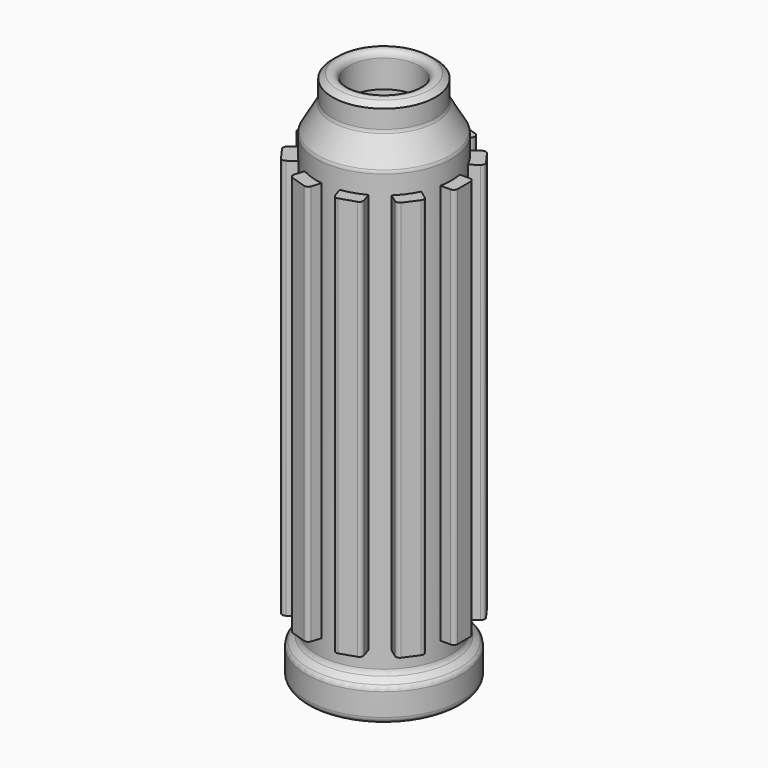
from build123d import *

# Parameters (mm, degrees)
F2_R            = 1.6
F4_W            = 6
F4_H            = 100
F5_COPIES_COUNT = 10
F6_R            = 1
F6_2_R          = 1
F6_3_R          = 1
F6_4_R          = 1
F6_5_R          = 1
F6_6_R          = 1
F6_7_R          = 1
F6_8_R          = 1
F6_9_R          = 1
F6_10_R         = 1


# Not quite as in the source:
# - a feature of the source that left no trace in its solid (it failed there, or was rolled back) is left out
# - a pattern or mirror of a feature is missing from the dataset's text; its kind, count and spacing are read off the source's solid


with BuildPart() as f1:
    # F0 (on Front) → F1 (revolve)
    with BuildSketch(Plane.XZ):
        with BuildLine():
            Line((10.75, 125), (10.75, 0))
            Line((10.75, 0), (19.325, 0))
            Line((19.325, 0), (19.325, 8))
            Line((19.325, 8), (16.7893237613, 10.1276849967))
            Line((16.7893237613, 10.1276849967), (16.7893237613, 120.1276849967))
            Line((16.7893237613, 120.1276849967), (12.8215908442, 127))
            Line((12.8215908442, 127), (12.8215908442, 132))
            ThreePointArc((12.8215908442, 132), (10.860884629, 133.5551954835), (8.8174703872, 135))
            Line((8.8174703872, 135), (8.8174703872, 125))
            Line((8.8174703872, 125), (10.75, 125))
        make_face()
    revolve(axis=Axis((0, 0, 18.1783709021), (0, 0, 1)))

    # F2
    f2_edges = [f1.edges().sort_by_distance(p)[0] for p in [
        (-8.81747, 0, 135),
        (-12.821591, 0, 127),
        (-16.789324, 0, 120.127685),
        (-16.789324, 0, 10.127685),
        (-19.325, 0, 8),
        (-19.325, 0, 0),
    ]]
    fillet(f2_edges, radius=F2_R)


with BuildPart() as f5:
    # F4 (on offset) → F5 (new body, up to the next surface of F1)
    with BuildSketch(Plane.YZ.offset(20)):
        with Locations((0, 65)):
            Rectangle(F4_W, F4_H)
    extrude(until=Until.NEXT, target=f1.part, dir=(-1, 0, 0))


with BuildPart() as f5_copies_1:
    # F5_copies: instance of F5
    add(f5.part.rotate(Axis((0, 0, 0), (0, 0, 1)), 1 * 360 / F5_COPIES_COUNT))

    # F6#2
    f6_2_edges = [f5_copies_1.edges().sort_by_distance(p)[0] for p in [
        (17.943696, 9.328654, 65),
        (14.416984, 14.182756, 65),
    ]]
    fillet(f6_2_edges, radius=F6_2_R)


with BuildPart() as f5_copies_2:
    # F5_copies: instance of F5
    add(f5.part.rotate(Axis((0, 0, 0), (0, 0, 1)), 2 * 360 / F5_COPIES_COUNT))

    # F6#3
    f6_3_edges = [f5_copies_2.edges().sort_by_distance(p)[0] for p in [
        (9.033509, 18.094079, 65),
        (3.32717, 19.948181, 65),
    ]]
    fillet(f6_3_edges, radius=F6_3_R)


with BuildPart() as f5_copies_3:
    # F5_copies: instance of F5
    add(f5.part.rotate(Axis((0, 0, 0), (0, 0, 1)), 3 * 360 / F5_COPIES_COUNT))

    # F6#4
    f6_4_edges = [f5_copies_3.edges().sort_by_distance(p)[0] for p in [
        (-3.32717, 19.948181, 65),
        (-9.033509, 18.094079, 65),
    ]]
    fillet(f6_4_edges, radius=F6_4_R)


with BuildPart() as f5_copies_4:
    # F5_copies: instance of F5
    add(f5.part.rotate(Axis((0, 0, 0), (0, 0, 1)), 4 * 360 / F5_COPIES_COUNT))

    # F6#5
    f6_5_edges = [f5_copies_4.edges().sort_by_distance(p)[0] for p in [
        (-14.416984, 14.182756, 65),
        (-17.943696, 9.328654, 65),
    ]]
    fillet(f6_5_edges, radius=F6_5_R)


with BuildPart() as f5_copies_5:
    # F5_copies: instance of F5
    add(f5.part.rotate(Axis((0, 0, 0), (0, 0, 1)), 5 * 360 / F5_COPIES_COUNT))

    # F6#6
    f6_6_edges = [f5_copies_5.edges().sort_by_distance(p)[0] for p in [
        (-20, 3, 65),
        (-20, -3, 65),
    ]]
    fillet(f6_6_edges, radius=F6_6_R)


with BuildPart() as f5_copies_6:
    # F5_copies: instance of F5
    add(f5.part.rotate(Axis((0, 0, 0), (0, 0, 1)), 6 * 360 / F5_COPIES_COUNT))

    # F6#7
    f6_7_edges = [f5_copies_6.edges().sort_by_distance(p)[0] for p in [
        (-17.943696, -9.328654, 65),
        (-14.416984, -14.182756, 65),
    ]]
    fillet(f6_7_edges, radius=F6_7_R)


with BuildPart() as f5_copies_7:
    # F5_copies: instance of F5
    add(f5.part.rotate(Axis((0, 0, 0), (0, 0, 1)), 7 * 360 / F5_COPIES_COUNT))

    # F6#8
    f6_8_edges = [f5_copies_7.edges().sort_by_distance(p)[0] for p in [
        (-9.033509, -18.094079, 65),
        (-3.32717, -19.948181, 65),
    ]]
    fillet(f6_8_edges, radius=F6_8_R)


with BuildPart() as f5_copies_8:
    # F5_copies: instance of F5
    add(f5.part.rotate(Axis((0, 0, 0), (0, 0, 1)), 8 * 360 / F5_COPIES_COUNT))

    # F6#9
    f6_9_edges = [f5_copies_8.edges().sort_by_distance(p)[0] for p in [
        (3.32717, -19.948181, 65),
        (9.033509, -18.094079, 65),
    ]]
    fillet(f6_9_edges, radius=F6_9_R)


with BuildPart() as f5_copies_9:
    # F5_copies: instance of F5
    add(f5.part.rotate(Axis((0, 0, 0), (0, 0, 1)), 9 * 360 / F5_COPIES_COUNT))

    # F6#10
    f6_10_edges = [f5_copies_9.edges().sort_by_distance(p)[0] for p in [
        (14.416984, -14.182756, 65),
        (17.943696, -9.328654, 65),
    ]]
    fillet(f6_10_edges, radius=F6_10_R)


with BuildPart() as f5_1:
    add(f5.part)

    # F6
    f6_edges = [f5_1.edges().sort_by_distance(p)[0] for p in [
        (20, -3, 65),
        (20, 3, 65),
    ]]
    fillet(f6_edges, radius=F6_R)


solid = Compound([f1.part, f5_copies_1.part, f5_copies_2.part, f5_copies_3.part, f5_copies_4.part, f5_copies_5.part, f5_copies_6.part, f5_copies_7.part, f5_copies_8.part, f5_copies_9.part, f5_1.part])
